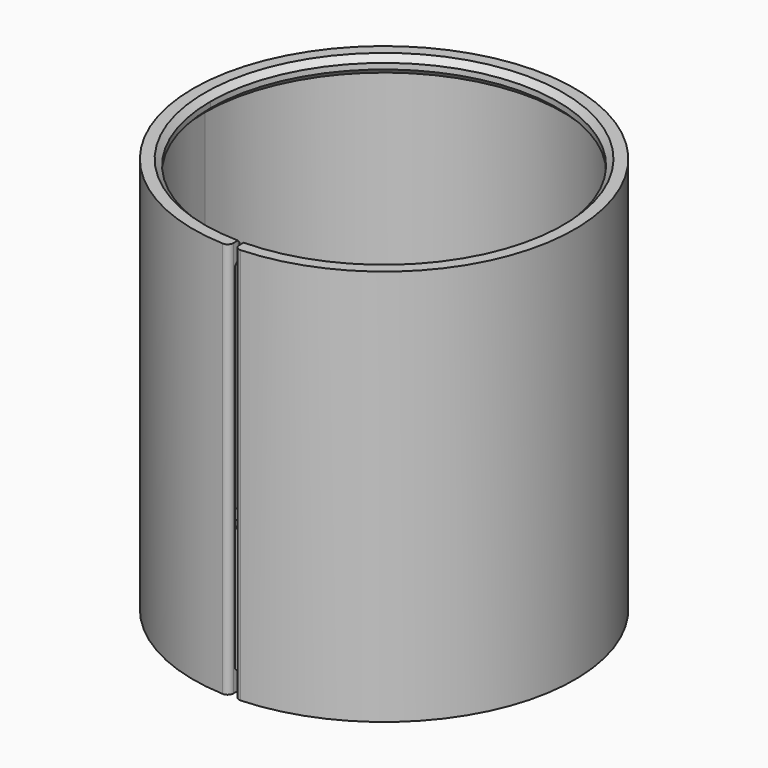
from build123d import *

# Parameters (mm, degrees)
F2_W     = 1
F2_H     = 40
F3_DEPTH = 68.601
F4_R     = 0.99999


# Not quite as in the source:
# - a fillet or chamfer is up to 0.001 mm smaller than in the source, because OpenCascade refuses the exact size


with BuildPart() as f1:
    # F0 (on Front) → F1 (revolve)
    with BuildSketch(Plane.XZ):
        Polygon((-33, 34.3), (-33, 0), (-31, 0), (-31, 31.3), (-30, 32.3), (-30, 33.3), (-31, 34.3), align=None)
        Polygon((-31, 0), (-33, 0), (-33, -34.3), (-31, -34.3), (-30, -33.3), (-30, -32.3), (-31, -31.3), align=None)
    revolve(axis=Axis((0, 0, 17.15), (0, 0, 1)))

    # F2 (on face) → F3 (cut, through all)
    with BuildSketch(Plane.XY.offset(34.3)):
        with Locations((0, -20)):
            Rectangle(F2_W, F2_H)
    extrude(amount=-F3_DEPTH, mode=Mode.SUBTRACT)

    # F4 (radius 1 in the source; OpenCascade refuses exactly that, so slightly less here)
    f4_edges = [f1.edges().sort_by_distance(p)[0] for p in [
        (-0.5, -32.996212, 0),
        (-0.5, -30.995967, 0),
        (-0.5, -29.995833, 32.8),
        (-0.5, -29.995833, -32.8),
        (0.5, -29.995833, -32.8),
        (0.5, -30.995967, 0),
        (0.5, -29.995833, 32.8),
        (0.5, -32.996212, 0),
    ]]
    fillet(f4_edges, radius=F4_R)


solid = f1.part
